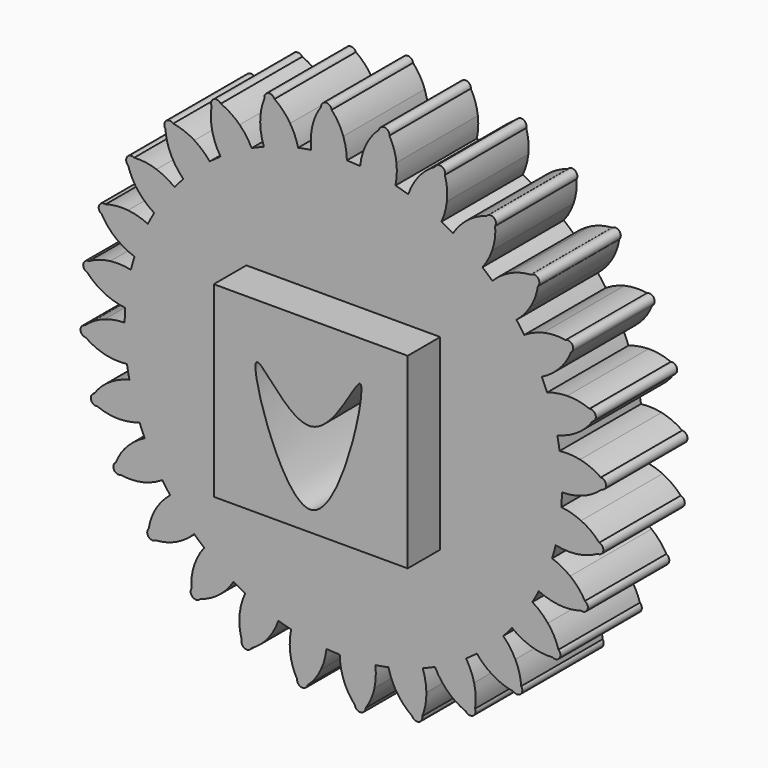
from build123d import *

# Parameters (mm, degrees)
F0_W     = 47.6354919374
F0_H     = 45.9833927453
F1_DEPTH = 25
F2_COUNT = 28
F3_DEPTH = 35


with BuildPart() as f1:
    # F0 (on Front) → F1 (new body)
    with BuildSketch(Plane.XZ):
        with BuildLine():
            ThreePointArc((-7.8842675869, 53.139290225), (-35.0884247435, -40.6785974441), (53.721, 0))
            ThreePointArc((53.721, 0), (38.2966086664, 37.6738052983), (0.8807473744, 53.7137796572))
            ThreePointArc((0.8807473744, 53.7137796572), (-3.5135215054, 53.6059792153), (-7.8842675869, 53.139290225))
        make_face()
        Rectangle(F0_W, F0_H, mode=Mode.SUBTRACT)
        with BuildLine():
            ThreePointArc((-7.8842675869, 53.139290225), (-3.5135215054, 53.6059792153), (0.8807473744, 53.7137796572))
            ThreePointArc((0.8807473744, 53.7137796572), (0.6444216491, 56.2301210228), (0, 58.674))
            ThreePointArc((0, 58.674), (-1.188832718, 61.1984634544), (-2.8564405638, 63.4357213824))
            ThreePointArc((-2.8564405638, 63.4357213824), (-4.2307667448, 64.5490269071), (-5.448019844, 63.2658603022))
            ThreePointArc((-5.448019844, 63.2658603022), (-6.8093403151, 60.8300759237), (-7.6584938023, 58.1720357962))
            ThreePointArc((-7.6584938023, 58.1720357962), (-7.9784121177, 55.6649506385), (-7.8842675869, 53.139290225))
        make_face()
    extrude(amount=F1_DEPTH)


with BuildPart() as f2_1:
    # F2: instance of F1
    add(f1.part.rotate(Axis((0, 0, 0), (0, 1, 0)), 1 * 360 / F2_COUNT))


with BuildPart() as f2_2:
    # F2: instance of F1
    add(f1.part.rotate(Axis((0, 0, 0), (0, 1, 0)), 2 * 360 / F2_COUNT))


with BuildPart() as f2_3:
    # F2: instance of F1
    add(f1.part.rotate(Axis((0, 0, 0), (0, 1, 0)), 3 * 360 / F2_COUNT))


with BuildPart() as f2_4:
    # F2: instance of F1
    add(f1.part.rotate(Axis((0, 0, 0), (0, 1, 0)), 4 * 360 / F2_COUNT))


with BuildPart() as f2_5:
    # F2: instance of F1
    add(f1.part.rotate(Axis((0, 0, 0), (0, 1, 0)), 5 * 360 / F2_COUNT))


with BuildPart() as f2_6:
    # F2: instance of F1
    add(f1.part.rotate(Axis((0, 0, 0), (0, 1, 0)), 6 * 360 / F2_COUNT))


with BuildPart() as f2_7:
    # F2: instance of F1
    add(f1.part.rotate(Axis((0, 0, 0), (0, 1, 0)), 7 * 360 / F2_COUNT))


with BuildPart() as f2_8:
    # F2: instance of F1
    add(f1.part.rotate(Axis((0, 0, 0), (0, 1, 0)), 8 * 360 / F2_COUNT))


with BuildPart() as f2_9:
    # F2: instance of F1
    add(f1.part.rotate(Axis((0, 0, 0), (0, 1, 0)), 9 * 360 / F2_COUNT))


with BuildPart() as f2_10:
    # F2: instance of F1
    add(f1.part.rotate(Axis((0, 0, 0), (0, 1, 0)), 10 * 360 / F2_COUNT))


with BuildPart() as f2_11:
    # F2: instance of F1
    add(f1.part.rotate(Axis((0, 0, 0), (0, 1, 0)), 11 * 360 / F2_COUNT))


with BuildPart() as f2_12:
    # F2: instance of F1
    add(f1.part.rotate(Axis((0, 0, 0), (0, 1, 0)), 12 * 360 / F2_COUNT))


with BuildPart() as f2_13:
    # F2: instance of F1
    add(f1.part.rotate(Axis((0, 0, 0), (0, 1, 0)), 13 * 360 / F2_COUNT))


with BuildPart() as f2_14:
    # F2: instance of F1
    add(f1.part.rotate(Axis((0, 0, 0), (0, 1, 0)), 14 * 360 / F2_COUNT))


with BuildPart() as f2_15:
    # F2: instance of F1
    add(f1.part.rotate(Axis((0, 0, 0), (0, 1, 0)), 15 * 360 / F2_COUNT))


with BuildPart() as f2_16:
    # F2: instance of F1
    add(f1.part.rotate(Axis((0, 0, 0), (0, 1, 0)), 16 * 360 / F2_COUNT))


with BuildPart() as f2_17:
    # F2: instance of F1
    add(f1.part.rotate(Axis((0, 0, 0), (0, 1, 0)), 17 * 360 / F2_COUNT))


with BuildPart() as f2_18:
    # F2: instance of F1
    add(f1.part.rotate(Axis((0, 0, 0), (0, 1, 0)), 18 * 360 / F2_COUNT))


with BuildPart() as f2_19:
    # F2: instance of F1
    add(f1.part.rotate(Axis((0, 0, 0), (0, 1, 0)), 19 * 360 / F2_COUNT))


with BuildPart() as f2_20:
    # F2: instance of F1
    add(f1.part.rotate(Axis((0, 0, 0), (0, 1, 0)), 20 * 360 / F2_COUNT))


with BuildPart() as f2_21:
    # F2: instance of F1
    add(f1.part.rotate(Axis((0, 0, 0), (0, 1, 0)), 21 * 360 / F2_COUNT))


with BuildPart() as f2_22:
    # F2: instance of F1
    add(f1.part.rotate(Axis((0, 0, 0), (0, 1, 0)), 22 * 360 / F2_COUNT))


with BuildPart() as f2_23:
    # F2: instance of F1
    add(f1.part.rotate(Axis((0, 0, 0), (0, 1, 0)), 23 * 360 / F2_COUNT))


with BuildPart() as f2_24:
    # F2: instance of F1
    add(f1.part.rotate(Axis((0, 0, 0), (0, 1, 0)), 24 * 360 / F2_COUNT))


with BuildPart() as f2_25:
    # F2: instance of F1
    add(f1.part.rotate(Axis((0, 0, 0), (0, 1, 0)), 25 * 360 / F2_COUNT))


with BuildPart() as f2_26:
    # F2: instance of F1
    add(f1.part.rotate(Axis((0, 0, 0), (0, 1, 0)), 26 * 360 / F2_COUNT))


with BuildPart() as f2_27:
    # F2: instance of F1
    add(f1.part.rotate(Axis((0, 0, 0), (0, 1, 0)), 27 * 360 / F2_COUNT))


with BuildPart() as f1_1:
    add(f1.part)

    add(f2_1.part)  # F3 merges F2_1

    add(f2_2.part)  # F3 merges F2_2

    add(f2_3.part)  # F3 merges F2_3

    add(f2_4.part)  # F3 merges F2_4

    add(f2_5.part)  # F3 merges F2_5

    add(f2_6.part)  # F3 merges F2_6

    add(f2_7.part)  # F3 merges F2_7

    add(f2_8.part)  # F3 merges F2_8

    add(f2_9.part)  # F3 merges F2_9

    add(f2_10.part)  # F3 merges F2_10

    add(f2_11.part)  # F3 merges F2_11

    add(f2_12.part)  # F3 merges F2_12

    add(f2_13.part)  # F3 merges F2_13

    add(f2_14.part)  # F3 merges F2_14

    add(f2_15.part)  # F3 merges F2_15

    add(f2_16.part)  # F3 merges F2_16

    add(f2_17.part)  # F3 merges F2_17

    add(f2_18.part)  # F3 merges F2_18

    add(f2_19.part)  # F3 merges F2_19

    add(f2_20.part)  # F3 merges F2_20

    add(f2_21.part)  # F3 merges F2_21

    add(f2_22.part)  # F3 merges F2_22

    add(f2_23.part)  # F3 merges F2_23

    add(f2_24.part)  # F3 merges F2_24

    add(f2_25.part)  # F3 merges F2_25

    add(f2_26.part)  # F3 merges F2_26

    add(f2_27.part)  # F3 merges F2_27
    # F0 (on Front) → F3 (join)
    with BuildSketch(Plane.XZ):
        Rectangle(F0_W, F0_H)
        with BuildLine():
            add(Edge.make_bspline(
                [(0, 0), (5.977603906, 0.5568687699), (18.3287253509, 32.878632874), (1.3080243344, -45.552466636), (-20.882127807, 26.5649050766), (-5.716139316, -0.5325109391), (0, 0)],
                knots=[0, 0, 0, 0, 0.2160315095, 0.5111237473, 0.7934178603, 1, 1, 1, 1], degree=3))
        make_face(mode=Mode.SUBTRACT)
    extrude(amount=F3_DEPTH)


solid = f1_1.part
